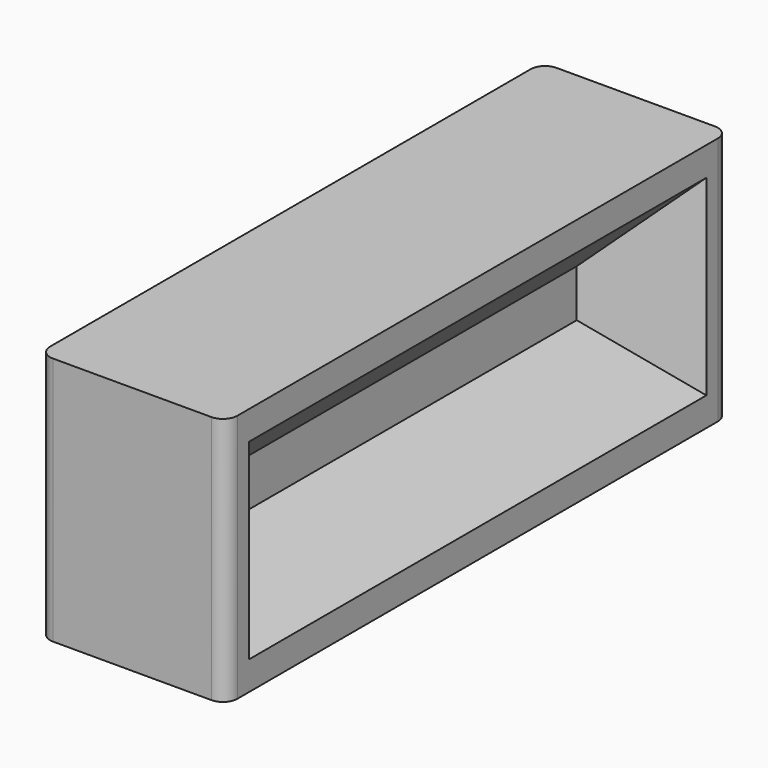
from build123d import *

# Parameters (mm, degrees)
F0_W     = 13
F0_H     = 43.7
F1_DEPTH = 17.3
F2_R     = 1
F3_W     = 39.7
F3_H     = 13.3
F5_DEPTH = 5
F4_W     = 39.7
F4_H     = 13.3
F6_DEPTH = 5
F7_SIZE  = 4.99999


# Not quite as in the source:
# - a fillet or chamfer is up to 0.001 mm smaller than in the source, because OpenCascade refuses the exact size


with BuildPart() as f1:
    # F0 (on Top) → F1 (new body)
    with BuildSketch(Plane.XY):
        Rectangle(F0_W, F0_H)
    extrude(amount=F1_DEPTH)

    # F2
    f2_edges = [f1.edges().sort_by_distance(p)[0] for p in [
        (-6.5, 21.85, 8.65),
        (6.5, 21.85, 8.65),
        (-6.5, -21.85, 8.65),
        (6.5, -21.85, 8.65),
    ]]
    fillet(f2_edges, radius=F2_R)

    # F3 (on face) → F5 (cut)
    with BuildSketch(Plane.YZ.offset(6.5)):
        with Locations((0, 8.65)):
            Rectangle(F3_W, F3_H)
    extrude(amount=-F5_DEPTH, mode=Mode.SUBTRACT)

    # F4 (on face) → F6 (cut)
    with BuildSketch(Plane(origin=(-6.5, 0, 0), x_dir=(0, -1, 0), z_dir=(-1, 0, 0))):
        with Locations((0, 8.65)):
            Rectangle(F4_W, F4_H)
    extrude(amount=-F6_DEPTH, mode=Mode.SUBTRACT)

    # F7 (size 5 in the source; OpenCascade refuses exactly that, so slightly less here)
    f7_edges = [f1.edges().sort_by_distance(p)[0] for p in [
        (-1.5, 0, 2),
        (-1.5, 19.85, 8.65),
        (-1.5, 0, 15.3),
        (-1.5, -19.85, 8.65),
        (1.5, 19.85, 8.65),
        (1.5, 0, 2),
        (1.5, -19.85, 8.65),
        (1.5, 0, 15.3),
    ]]
    chamfer(f7_edges, length=F7_SIZE)


solid = f1.part
